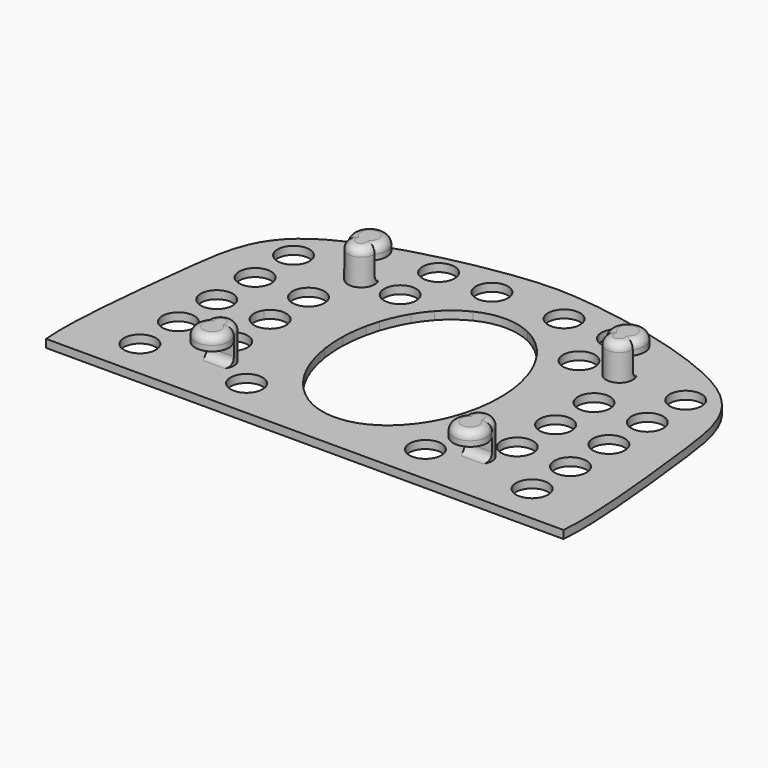
from build123d import *

# Parameters (mm, degrees)
F0_R     = 3
F1_DEPTH = 1.5
F2_DEPTH = 8
F3_START = 5.5
F3_DEPTH = 2.5
F4_R     = 1.5


# Not quite as in the source:
# - a feature names something its author has since deleted; it is built from what else it names


with BuildPart() as f1:
    # F0 (on Top) → F1 (new body)
    with BuildSketch(Plane.XY):
        with BuildLine():
            add(Edge.make_bspline(
                [(-48.5, 0), (-49.1826629275, 6.5220924307), (-46.4556473513, 31.1291488734), (-43.6314940449, 52.639490161), (-8.3544173495, 59.0869885527), (0, 59)],
                knots=[0, 0, 0, 0, 0.3361084439, 0.6157630382, 1, 1, 1, 1], degree=3))
            Line((-48.5, 0), (0, 0))
            Line((0, 0), (0, 7))
            add(Edge.make_bspline(
                [(-3.7818023708, 7.646081266), (-1.9219444937, 7), (0, 7)],
                knots=[2.8867220875, 2.8867220875, 2.8867220875, 3.1415926536, 3.1415926536, 3.1415926536], degree=2, weights=[1, 0.9918911071, 1]))
            ThreePointArc((-3.7818023708, 7.646081266), (-3.7686227128, 7.4841819242), (-3.7642251961, 7.32180655))
            ThreePointArc((-3.7642251961, 7.32180655), (-8.4004272511, 4.807280186), (-7.9794537529, 10.0646553528))
            add(Edge.make_bspline(
                [(-11.709371247, 14.5), (-10.1254261893, 11.8622043427), (-7.9794537529, 10.0646553528)],
                knots=[2.2459278597, 2.2459278597, 2.2459278597, 2.5806748551, 2.5806748551, 2.5806748551], degree=2, weights=[1, 0.9860257247, 1]))
            Line((-11.709371247, 14.5), (-14.3807359693, 14.5))
            ThreePointArc((-14.3807359693, 14.5), (-16.7642251961, 13.32180655), (-19.1477144229, 14.5))
            Line((-19.1477144229, 14.5), (-24.3807359693, 14.5))
            ThreePointArc((-24.3807359693, 14.5), (-26.7642251961, 13.32180655), (-29.1477144229, 14.5))
            Line((-29.1477144229, 14.5), (-30, 14.5))
            Line((-30, 14.5), (-30, 27))
            Line((-30, 27), (-30, 39.5))
            Line((-30, 39.5), (-11.709371247, 39.5))
            add(Edge.make_bspline(
                [(-9.6061077156, 42.360711474), (-10.7657200353, 41.0714933142), (-11.709371247, 39.5)],
                knots=[0.6950283076, 0.6950283076, 0.6950283076, 0.8956647939, 0.8956647939, 0.8956647939], degree=2, weights=[1, 0.9949723436, 1]))
            ThreePointArc((-9.6061077156, 42.360711474), (-8.586457627, 45.7049701969), (-5.0918610257, 45.8124285771))
            add(Edge.make_bspline(
                [(0, 47), (-2.6238301557, 47), (-5.0918610257, 45.8124285771)],
                knots=[0, 0, 0, 0.3463399866, 0.3463399866, 0.3463399866], degree=2, weights=[1, 0.9850435089, 1]))
            Line((0, 47), (0, 54))
            Line((0, 54), (0, 59))
        make_face()
        with Locations((-36.7642251961, 7.32180655)):
            Circle(F0_R, mode=Mode.SUBTRACT)
        with Locations((-16.7642251961, 7.32180655)):
            Circle(F0_R, mode=Mode.SUBTRACT)
        with BuildLine():
            ThreePointArc((-21.6969395429, 10.5), (-24.1969395429, 5.356110991), (-26.6969395429, 10.5))
            ThreePointArc((-26.6969395429, 10.5), (-24.1969395429, 13), (-21.6969395429, 10.5))
        make_face(mode=Mode.SUBTRACT)
        with Locations((-36.7642251961, 16.32180655)):
            Circle(F0_R, mode=Mode.SUBTRACT)
        with Locations((-36.7642251961, 25.32180655)):
            Circle(F0_R, mode=Mode.SUBTRACT)
        with Locations((-36.7642251961, 34.32180655)):
            Circle(F0_R, mode=Mode.SUBTRACT)
        with Locations((-36.7642251961, 43.32180655)):
            Circle(F0_R, mode=Mode.SUBTRACT)
        with Locations((-16.7642251961, 43.32180655)):
            Circle(F0_R, mode=Mode.SUBTRACT)
        with BuildLine():
            ThreePointArc((-21.6969395429, 43.5), (-24.1969395429, 41), (-26.6969395429, 43.5))
            ThreePointArc((-26.6969395429, 43.5), (-24.1969395429, 48.643889009), (-21.6969395429, 43.5))
        make_face(mode=Mode.SUBTRACT)
        with Locations((-16.7642251961, 52.32180655)):
            Circle(F0_R, mode=Mode.SUBTRACT)
        with Locations((-6.7642251961, 52.32180655)):
            Circle(F0_R, mode=Mode.SUBTRACT)
        with BuildLine():
            Line((0, 7), (0, 0))
            Line((0, 0), (48.5, 0))
            add(Edge.make_bspline(
                [(48.5, 0), (49.1826629275, 6.5220924307), (46.4556473513, 31.1291488734), (43.6314940449, 52.639490161), (8.3544173495, 59.0869885527), (0, 59)],
                knots=[0, 0, 0, 0, 0.3361084439, 0.6157630382, 1, 1, 1, 1], degree=3))
            Line((0, 59), (0, 54))
            Line((0, 54), (0, 47))
            add(Edge.make_bspline(
                [(5.0918610257, 45.8124285771), (2.6238301557, 47), (0, 47)],
                knots=[5.9368453206, 5.9368453206, 5.9368453206, 6.2831853072, 6.2831853072, 6.2831853072], degree=2, weights=[1, 0.9850435089, 1]))
            ThreePointArc((5.0918610257, 45.8124285771), (8.1754139661, 45.9691724589), (9.7642251961, 43.32180655))
            ThreePointArc((9.7642251961, 43.32180655), (9.7244319084, 42.8347991366), (9.6061077156, 42.360711474))
            add(Edge.make_bspline(
                [(11.709371247, 39.5), (10.7657200353, 41.0714933142), (9.6061077156, 42.360711474)],
                knots=[5.3875205133, 5.3875205133, 5.3875205133, 5.5881569996, 5.5881569996, 5.5881569996], degree=2, weights=[1, 0.9949723436, 1]))
            Line((11.709371247, 39.5), (30, 39.5))
            Line((30, 39.5), (30, 14.5))
            Line((30, 14.5), (29.1477144229, 14.5))
            ThreePointArc((29.1477144229, 14.5), (26.7642251961, 13.32180655), (24.3807359693, 14.5))
            Line((24.3807359693, 14.5), (19.1477144229, 14.5))
            ThreePointArc((19.1477144229, 14.5), (16.7642251961, 13.32180655), (14.3807359693, 14.5))
            Line((14.3807359693, 14.5), (11.709371247, 14.5))
            add(Edge.make_bspline(
                [(7.9794537529, 10.0646553528), (10.1254261893, 11.8622043427), (11.709371247, 14.5)],
                knots=[3.7025104521, 3.7025104521, 3.7025104521, 4.0372574474, 4.0372574474, 4.0372574474], degree=2, weights=[1, 0.9860257247, 1]))
            ThreePointArc((7.9794537529, 10.0646553528), (9.2787515601, 8.958008605), (9.7642251961, 7.32180655))
            ThreePointArc((9.7642251961, 7.32180655), (6.6018498219, 4.3262040667), (3.7818023708, 7.646081266))
            add(Edge.make_bspline(
                [(0, 7), (1.9219444937, 7), (3.7818023708, 7.646081266)],
                knots=[3.1415926536, 3.1415926536, 3.1415926536, 3.3964632197, 3.3964632197, 3.3964632197], degree=2, weights=[1, 0.9918911071, 1]))
        make_face()
        with Locations((16.7642251961, 7.32180655)):
            Circle(F0_R, mode=Mode.SUBTRACT)
        with BuildLine():
            ThreePointArc((21.6969395429, 10.5), (24.1969395429, 13), (26.6969395429, 10.5))
            ThreePointArc((26.6969395429, 10.5), (24.1969395429, 5.356110991), (21.6969395429, 10.5))
        make_face(mode=Mode.SUBTRACT)
        with Locations((36.7642251961, 7.32180655)):
            Circle(F0_R, mode=Mode.SUBTRACT)
        with Locations((36.7642251961, 16.32180655)):
            Circle(F0_R, mode=Mode.SUBTRACT)
        with Locations((36.7642251961, 25.32180655)):
            Circle(F0_R, mode=Mode.SUBTRACT)
        with Locations((16.7642251961, 43.32180655)):
            Circle(F0_R, mode=Mode.SUBTRACT)
        with Locations((36.7642251961, 34.32180655)):
            Circle(F0_R, mode=Mode.SUBTRACT)
        with Locations((36.7642251961, 43.32180655)):
            Circle(F0_R, mode=Mode.SUBTRACT)
        with BuildLine():
            ThreePointArc((21.6969395429, 43.5), (24.1969395429, 48.643889009), (26.6969395429, 43.5))
            ThreePointArc((26.6969395429, 43.5), (24.1969395429, 41), (21.6969395429, 43.5))
        make_face(mode=Mode.SUBTRACT)
        with Locations((6.7642251961, 52.32180655)):
            Circle(F0_R, mode=Mode.SUBTRACT)
        with Locations((16.7642251961, 52.32180655)):
            Circle(F0_R, mode=Mode.SUBTRACT)
        with BuildLine():
            add(Edge.make_bspline(
                [(-11.709371247, 39.5), (-12.9990529265, 37.3522507981), (-13.805873476, 34.819958234)],
                knots=[0.8956647939, 0.8956647939, 0.8956647939, 1.1690807583, 1.1690807583, 1.1690807583], degree=2, weights=[1, 0.9906700081, 1]))
            Line((-11.709371247, 39.5), (-30, 39.5))
            Line((-30, 39.5), (-30, 27))
            Line((-30, 27), (-29.2509231561, 27))
            ThreePointArc((-29.2509231561, 27), (-26.7642251961, 28.32180655), (-24.2775272361, 27))
            Line((-24.2775272361, 27), (-19.2509231561, 27))
            ThreePointArc((-19.2509231561, 27), (-17.2779990588, 28.277485223), (-14.9897092621, 27.7407098552))
            add(Edge.make_bspline(
                [(-14.4368123202, 32.4288857104), (-14.9233295117, 30.1288410124), (-14.9897092621, 27.7407098552)],
                knots=[1.2959029843, 1.2959029843, 1.2959029843, 1.5337523623, 1.5337523623, 1.5337523623], degree=2, weights=[1, 0.9929367897, 1]))
            ThreePointArc((-14.4368123202, 32.4288857104), (-19.6649378317, 35.087225524), (-13.805873476, 34.819958234))
        make_face()
        with Locations((-26.7642251961, 34.32180655)):
            Circle(F0_R, mode=Mode.SUBTRACT)
        with BuildLine():
            add(Edge.make_bspline(
                [(11.709371247, 14.5), (14.0054504395, 18.3237359897), (14.7164204545, 23.1294343781)],
                knots=[4.0372574474, 4.0372574474, 4.0372574474, 4.5176318311, 4.5176318311, 4.5176318311], degree=2, weights=[1, 0.9712934618, 1]))
            Line((11.709371247, 14.5), (14.3807359693, 14.5))
            ThreePointArc((14.3807359693, 14.5), (15.8025775684, 19.1635021425), (19.7642251961, 16.32180655))
            ThreePointArc((19.7642251961, 16.32180655), (19.6059207886, 15.3601589224), (19.1477144229, 14.5))
            Line((19.1477144229, 14.5), (24.3807359693, 14.5))
            ThreePointArc((24.3807359693, 14.5), (25.8025775684, 19.1635021425), (29.7642251961, 16.32180655))
            ThreePointArc((29.7642251961, 16.32180655), (29.6059207886, 15.3601589224), (29.1477144229, 14.5))
            Line((29.1477144229, 14.5), (30, 14.5))
            Line((30, 14.5), (30, 39.5))
            Line((30, 39.5), (11.709371247, 39.5))
            add(Edge.make_bspline(
                [(13.805873476, 34.819958234), (12.9990529265, 37.3522507981), (11.709371247, 39.5)],
                knots=[5.1141045489, 5.1141045489, 5.1141045489, 5.3875205133, 5.3875205133, 5.3875205133], degree=2, weights=[1, 0.9906700081, 1]))
            ThreePointArc((13.805873476, 34.819958234), (17.0141700297, 37.3113763485), (19.7642251961, 34.32180655))
            ThreePointArc((19.7642251961, 34.32180655), (17.7686557244, 31.4949497595), (14.4368123202, 32.4288857104))
            add(Edge.make_bspline(
                [(14.9897092621, 27.7407098552), (14.9233295117, 30.1288410124), (14.4368123202, 32.4288857104)],
                knots=[4.7494329449, 4.7494329449, 4.7494329449, 4.9872823229, 4.9872823229, 4.9872823229], degree=2, weights=[1, 0.9929367897, 1]))
            ThreePointArc((14.9897092621, 27.7407098552), (18.1200371665, 27.9979556305), (19.7642251961, 25.32180655))
            ThreePointArc((19.7642251961, 25.32180655), (17.9593372777, 22.5701330388), (14.7164204545, 23.1294343781))
        make_face()
        with Locations((26.7642251961, 25.32180655)):
            Circle(F0_R, mode=Mode.SUBTRACT)
        with Locations((26.7642251961, 34.32180655)):
            Circle(F0_R, mode=Mode.SUBTRACT)
        with BuildLine():
            Line((-14.3807359693, 14.5), (-11.709371247, 14.5))
            add(Edge.make_bspline(
                [(-14.7164204545, 23.1294343781), (-14.0054504395, 18.3237359897), (-11.709371247, 14.5)],
                knots=[1.7655534761, 1.7655534761, 1.7655534761, 2.2459278597, 2.2459278597, 2.2459278597], degree=2, weights=[1, 0.9712934618, 1]))
            ThreePointArc((-14.7164204545, 23.1294343781), (-18.7119100712, 23.0400257483), (-19.2509231561, 27))
            Line((-19.2509231561, 27), (-24.2775272361, 27))
            ThreePointArc((-24.2775272361, 27), (-23.8954193574, 26.1992762418), (-23.7642251961, 25.32180655))
            ThreePointArc((-23.7642251961, 25.32180655), (-27.6416948878, 22.4530007113), (-29.2509231561, 27))
            Line((-29.2509231561, 27), (-30, 27))
            Line((-30, 27), (-30, 14.5))
            Line((-30, 14.5), (-29.1477144229, 14.5))
            ThreePointArc((-29.1477144229, 14.5), (-27.7258728238, 19.1635021425), (-23.7642251961, 16.32180655))
            ThreePointArc((-23.7642251961, 16.32180655), (-23.9225296036, 15.3601589224), (-24.3807359693, 14.5))
            Line((-24.3807359693, 14.5), (-19.1477144229, 14.5))
            ThreePointArc((-19.1477144229, 14.5), (-17.7258728238, 19.1635021425), (-13.7642251961, 16.32180655))
            ThreePointArc((-13.7642251961, 16.32180655), (-13.9225296036, 15.3601589224), (-14.3807359693, 14.5))
        make_face()
        with BuildLine():
            ThreePointArc((-19.2509231561, 27), (-18.7119100712, 23.0400257483), (-14.7164204545, 23.1294343781))
            add(Edge.make_bspline(
                [(-15, 27), (-15, 25.0462490623), (-14.7164204545, 23.1294343781)],
                knots=[1.5707963268, 1.5707963268, 1.5707963268, 1.7655534761, 1.7655534761, 1.7655534761], degree=2, weights=[1, 0.9952624521, 1]))
            Line((-15, 27), (-19.2509231561, 27))
        make_face()
        with BuildLine():
            Line((-19.2509231561, 27), (-15, 27))
            add(Edge.make_bspline(
                [(-14.9897092621, 27.7407098552), (-15, 27.3704820121), (-15, 27)],
                knots=[1.5337523623, 1.5337523623, 1.5337523623, 1.5707963268, 1.5707963268, 1.5707963268], degree=2, weights=[1, 0.999828473, 1]))
            ThreePointArc((-14.9897092621, 27.7407098552), (-17.2779990588, 28.277485223), (-19.2509231561, 27))
        make_face()
        with BuildLine():
            add(Edge.make_bspline(
                [(-5.0918610257, 45.8124285771), (-7.5769690172, 44.616639955), (-9.6061077156, 42.360711474)],
                knots=[0.3463399866, 0.3463399866, 0.3463399866, 0.6950283076, 0.6950283076, 0.6950283076], degree=2, weights=[1, 0.9848405141, 1]))
            ThreePointArc((-5.0918610257, 45.8124285771), (-8.586457627, 45.7049701969), (-9.6061077156, 42.360711474))
        make_face()
        with BuildLine():
            ThreePointArc((9.7642251961, 43.32180655), (8.1754139661, 45.9691724589), (5.0918610257, 45.8124285771))
            add(Edge.make_bspline(
                [(9.6061077156, 42.360711474), (7.5769690172, 44.616639955), (5.0918610257, 45.8124285771)],
                knots=[5.5881569996, 5.5881569996, 5.5881569996, 5.9368453206, 5.9368453206, 5.9368453206], degree=2, weights=[1, 0.9848405141, 1]))
            ThreePointArc((9.6061077156, 42.360711474), (9.7244319084, 42.8347991366), (9.7642251961, 43.32180655))
        make_face()
        with BuildLine():
            ThreePointArc((-3.7642251961, 7.32180655), (-3.7686227128, 7.4841819242), (-3.7818023708, 7.646081266))
            add(Edge.make_bspline(
                [(-7.9794537529, 10.0646553528), (-6.020508703, 8.4237676899), (-3.7818023708, 7.646081266)],
                knots=[2.5806748551, 2.5806748551, 2.5806748551, 2.8867220875, 2.8867220875, 2.8867220875], degree=2, weights=[1, 0.9883147153, 1]))
            ThreePointArc((-7.9794537529, 10.0646553528), (-8.4004272511, 4.807280186), (-3.7642251961, 7.32180655))
        make_face()
        with BuildLine():
            add(Edge.make_bspline(
                [(3.7818023708, 7.646081266), (6.020508703, 8.4237676899), (7.9794537529, 10.0646553528)],
                knots=[3.3964632197, 3.3964632197, 3.3964632197, 3.7025104521, 3.7025104521, 3.7025104521], degree=2, weights=[1, 0.9883147153, 1]))
            ThreePointArc((3.7818023708, 7.646081266), (6.6018498219, 4.3262040667), (9.7642251961, 7.32180655))
            ThreePointArc((9.7642251961, 7.32180655), (9.2787515601, 8.958008605), (7.9794537529, 10.0646553528))
        make_face()
        with BuildLine():
            add(Edge.make_bspline(
                [(14.7164204545, 23.1294343781), (15.0543856332, 25.4138608382), (14.9897092621, 27.7407098552)],
                knots=[4.5176318311, 4.5176318311, 4.5176318311, 4.7494329449, 4.7494329449, 4.7494329449], degree=2, weights=[1, 0.9932910456, 1]))
            ThreePointArc((14.7164204545, 23.1294343781), (17.9593372777, 22.5701330388), (19.7642251961, 25.32180655))
            ThreePointArc((19.7642251961, 25.32180655), (18.1200371665, 27.9979556305), (14.9897092621, 27.7407098552))
        make_face()
        with BuildLine():
            add(Edge.make_bspline(
                [(-13.805873476, 34.819958234), (-14.1782769423, 33.6511301356), (-14.4368123202, 32.4288857104)],
                knots=[1.1690807583, 1.1690807583, 1.1690807583, 1.2959029843, 1.2959029843, 1.2959029843], degree=2, weights=[1, 0.997990189, 1]))
            ThreePointArc((-13.805873476, 34.819958234), (-19.6649378317, 35.087225524), (-14.4368123202, 32.4288857104))
        make_face()
        with BuildLine():
            ThreePointArc((19.7642251961, 34.32180655), (17.0141700297, 37.3113763485), (13.805873476, 34.819958234))
            add(Edge.make_bspline(
                [(14.4368123202, 32.4288857104), (14.1782769423, 33.6511301356), (13.805873476, 34.819958234)],
                knots=[4.9872823229, 4.9872823229, 4.9872823229, 5.1141045489, 5.1141045489, 5.1141045489], degree=2, weights=[1, 0.997990189, 1]))
            ThreePointArc((14.4368123202, 32.4288857104), (17.7686557244, 31.4949497595), (19.7642251961, 34.32180655))
        make_face()
        with BuildLine():
            Line((-19.1477144229, 14.5), (-14.3807359693, 14.5))
            ThreePointArc((-14.3807359693, 14.5), (-13.9225296036, 15.3601589224), (-13.7642251961, 16.32180655))
            ThreePointArc((-13.7642251961, 16.32180655), (-17.7258728238, 19.1635021425), (-19.1477144229, 14.5))
        make_face()
        with BuildLine():
            ThreePointArc((19.7642251961, 16.32180655), (15.8025775684, 19.1635021425), (14.3807359693, 14.5))
            Line((14.3807359693, 14.5), (19.1477144229, 14.5))
            ThreePointArc((19.1477144229, 14.5), (19.6059207886, 15.3601589224), (19.7642251961, 16.32180655))
        make_face()
        with BuildLine():
            ThreePointArc((-19.1477144229, 14.5), (-16.7642251961, 13.32180655), (-14.3807359693, 14.5))
            Line((-14.3807359693, 14.5), (-19.1477144229, 14.5))
        make_face()
        with BuildLine():
            Line((19.1477144229, 14.5), (14.3807359693, 14.5))
            ThreePointArc((14.3807359693, 14.5), (16.7642251961, 13.32180655), (19.1477144229, 14.5))
        make_face()
        with BuildLine():
            Line((-21.6969395429, 43.5), (-26.6969395429, 43.5))
            ThreePointArc((-26.6969395429, 43.5), (-24.1969395429, 41), (-21.6969395429, 43.5))
        make_face()
        with BuildLine():
            ThreePointArc((-21.6969395429, 43.5), (-24.1969395429, 48.643889009), (-26.6969395429, 43.5))
            Line((-26.6969395429, 43.5), (-21.6969395429, 43.5))
        make_face()
        with BuildLine():
            Line((21.6969395429, 43.5), (26.6969395429, 43.5))
            ThreePointArc((26.6969395429, 43.5), (24.1969395429, 48.643889009), (21.6969395429, 43.5))
        make_face()
        with BuildLine():
            ThreePointArc((21.6969395429, 43.5), (24.1969395429, 41), (26.6969395429, 43.5))
            Line((26.6969395429, 43.5), (21.6969395429, 43.5))
        make_face()
        with BuildLine():
            Line((21.6969395429, 10.5), (26.6969395429, 10.5))
            ThreePointArc((26.6969395429, 10.5), (24.1969395429, 13), (21.6969395429, 10.5))
        make_face()
        with BuildLine():
            ThreePointArc((21.6969395429, 10.5), (24.1969395429, 5.356110991), (26.6969395429, 10.5))
            Line((26.6969395429, 10.5), (21.6969395429, 10.5))
        make_face()
        with BuildLine():
            ThreePointArc((-21.6969395429, 10.5), (-24.1969395429, 13), (-26.6969395429, 10.5))
            Line((-26.6969395429, 10.5), (-21.6969395429, 10.5))
        make_face()
        with BuildLine():
            Line((-21.6969395429, 10.5), (-26.6969395429, 10.5))
            ThreePointArc((-26.6969395429, 10.5), (-24.1969395429, 5.356110991), (-21.6969395429, 10.5))
        make_face()
    extrude(amount=F1_DEPTH)

    # F0 (on Top) → F2 (join)
    with BuildSketch(Plane.XY):
        with BuildLine():
            Line((-21.6969395429, 43.5), (-26.6969395429, 43.5))
            ThreePointArc((-26.6969395429, 43.5), (-24.1969395429, 41), (-21.6969395429, 43.5))
        make_face()
        with BuildLine():
            ThreePointArc((-21.6969395429, 10.5), (-24.1969395429, 13), (-26.6969395429, 10.5))
            Line((-26.6969395429, 10.5), (-21.6969395429, 10.5))
        make_face()
        with BuildLine():
            Line((21.6969395429, 10.5), (26.6969395429, 10.5))
            ThreePointArc((26.6969395429, 10.5), (24.1969395429, 13), (21.6969395429, 10.5))
        make_face()
        with BuildLine():
            ThreePointArc((21.6969395429, 43.5), (24.1969395429, 41), (26.6969395429, 43.5))
            Line((26.6969395429, 43.5), (21.6969395429, 43.5))
        make_face()
    extrude(amount=F2_DEPTH)

    # F0 (on Top) → F3 (join)
    with BuildSketch(Plane.XY.offset(F3_START)):
        with BuildLine():
            Line((-21.6969395429, 10.5), (-26.6969395429, 10.5))
            ThreePointArc((-26.6969395429, 10.5), (-24.1969395429, 5.356110991), (-21.6969395429, 10.5))
        make_face()
        with BuildLine():
            ThreePointArc((21.6969395429, 10.5), (24.1969395429, 5.356110991), (26.6969395429, 10.5))
            Line((26.6969395429, 10.5), (21.6969395429, 10.5))
        make_face()
        with BuildLine():
            ThreePointArc((-21.6969395429, 43.5), (-24.1969395429, 48.643889009), (-26.6969395429, 43.5))
            Line((-26.6969395429, 43.5), (-21.6969395429, 43.5))
        make_face()
        with BuildLine():
            Line((21.6969395429, 43.5), (26.6969395429, 43.5))
            ThreePointArc((26.6969395429, 43.5), (24.1969395429, 48.643889009), (21.6969395429, 43.5))
        make_face()
    extrude(amount=F3_DEPTH)

    # F4
    f4_edges = [f1.edges().sort_by_distance(p)[0] for p in [
        (-24.19694, 41, 8),
        (-24.19694, 48.643889, 8),
        (-24.19694, 13, 8),
        (-24.19694, 5.356111, 8),
        (24.19694, 13, 8),
        (24.19694, 5.356111, 8),
        (24.19694, 41, 8),
        (24.19694, 48.643889, 8),
        (-24.19694, 43.5, 1.5),
        (24.19694, 43.5, 1.5),
        (24.19694, 10.5, 1.5),
        (-24.19694, 10.5, 1.5),
    ]]
    fillet(f4_edges, radius=F4_R)


solid = f1.part
